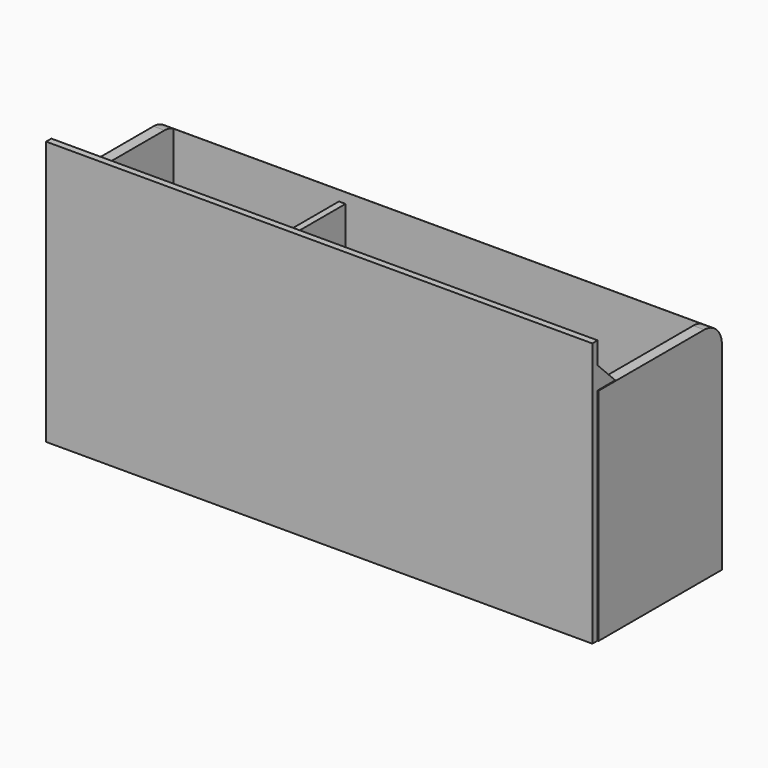
from build123d import *

# Parameters (mm, degrees)
F0_W         = 125
F0_H         = 35
F1_DEPTH     = 50
F2_T         = -2.5
F3_T1_DEPTH  = 150
F5_DEPTH     = 47
F6_W         = 123.983182013
F6_H         = 1.5
F7_DEPTH     = 60
F8_T4_DEPTH  = 136.8415969529
F8_T9_DEPTH  = 123.983182013
F8_T14_DEPTH = 136.8415969529


# Not quite as in the source:
# - a fillet or chamfer that OpenCascade refuses, or shapes differently, is made with other operations: its cross-section is extruded or revolved along the edge and cut away or added


with BuildPart() as f1:
    # F0 (on Top) → F1 (new body)
    with BuildSketch(Plane.XY):
        with Locations((-2.4887919426, 0.2054322337)):
            Rectangle(F0_W, F0_H)
    extrude(amount=F1_DEPTH)

    # F2
    f2_openings = [f1.faces().sort_by_distance(p)[0] for p in [
        (-2.488792, 0.205432, 50),
    ]]
    offset(amount=F2_T, openings=f2_openings)

    # F3: fillet of radius 5 on 1 edges, made by hand

    # F3_s2 → F3_t1 (cut)
    with BuildSketch(Plane.YZ.offset(-77.4887919426)):
        with BuildLine():
            ThreePointArc((17.7054322337, 45), (16.2409661396, 48.5355339059), (12.7054322337, 50))
            Line((12.7054322337, 50), (17.7054322337, 50))
            Line((17.7054322337, 50), (17.7054322337, 45))
        make_face()
    extrude(amount=F3_T1_DEPTH, mode=Mode.SUBTRACT)

    # F4 (on Top) → F5 (join)
    with BuildSketch(Plane.XY):
        Polygon((-23.4062603042, 15.2347357944), (-24.9062603042, 15.2233950794), (-24.9062603042, -14.9235967547), (-23.4062603042, -14.9009153247), align=None)
    extrude(amount=F5_DEPTH)

    # F6 (on Top) → F7 (join)
    with BuildSketch(Plane.XY):
        with Locations((-2.1866001189, -18.0445677663)):
            Rectangle(F6_W, F6_H)
    extrude(amount=F7_DEPTH)

    # F8: chamfer of 5 on 1 edges, made by hand


with BuildPart() as f8_tool2:
    # F8_s3 → F8_t4 (new body)
    with BuildSketch(Plane.YZ.offset(-64.1781911254)):
        Polygon((-12.2945677663, 50), (-17.2945677663, 55), (-17.2945677663, 50), align=None)
    extrude(amount=F8_T4_DEPTH)

    split(bisect_by=Plane.YZ.offset(-62.4887919426), keep=Keep.BOTTOM)


with BuildPart() as f1_1:
    add(f1.part)

    # F8_t1: union F8_tool2
    add(f8_tool2.part)


with BuildPart() as f8_tool7:
    # F8_s8 → F8_t9 (new body)
    with BuildSketch(Plane.YZ.offset(-64.1781911254)):
        Polygon((-12.2945677663, 50), (-17.2945677663, 55), (-17.2945677663, 50), align=None)
    extrude(amount=F8_T9_DEPTH)

    split(bisect_by=Plane.XZ.offset(14.7945677663), keep=Keep.TOP)


with BuildPart() as f1_2:
    add(f1_1.part)

    # F8_t6: union F8_tool7
    add(f8_tool7.part)


with BuildPart() as f8_tool12:
    # F8_s13 → F8_t14 (new body)
    with BuildSketch(Plane.YZ.offset(-77.0366060652)):
        Polygon((-12.2945677663, 50), (-17.2945677663, 55), (-17.2945677663, 50), align=None)
    extrude(amount=F8_T14_DEPTH)

    split(bisect_by=Plane.YZ.offset(57.5112080574), keep=Keep.TOP)


with BuildPart() as f1_3:
    add(f1_2.part)

    # F8_t11: union F8_tool12
    add(f8_tool12.part)


solid = f1_3.part
